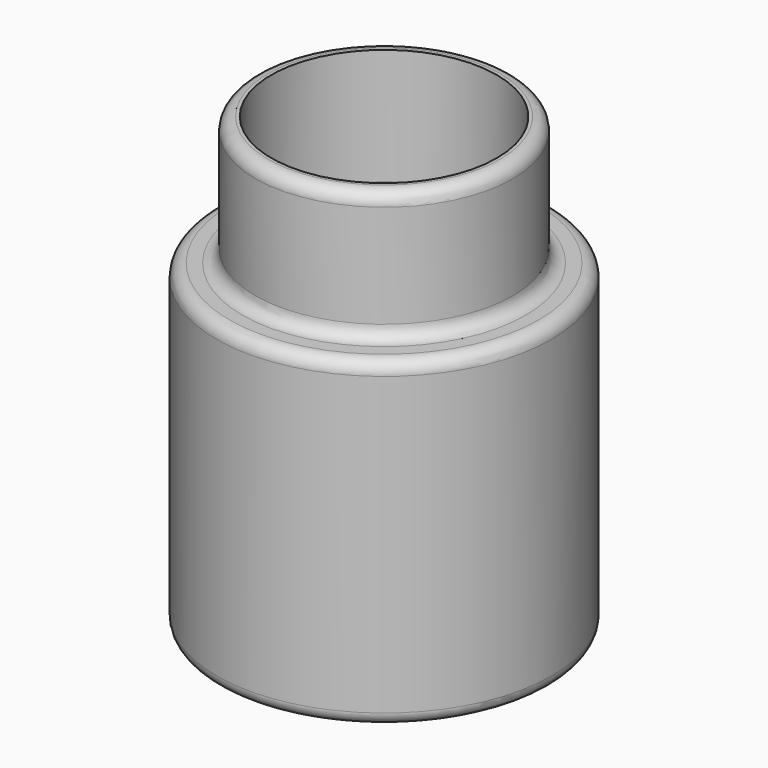
from build123d import *

# Parameters (mm, degrees)
F0_R     = 66.04
F1_DEPTH = 127
F2_R     = 5.08
F3_R     = 50.8
F3_R_2   = 44.45
F4_DEPTH = 50.8
F5_R     = 5.08
F6_T     = 2.54


# Not quite as in the source:
# - a shell that OpenCascade refuses in one call is made with other operations: the cavity is built on its own and cut out


with BuildPart() as f1:
    # F0 (on Top) → F1 (new body)
    with BuildSketch(Plane.XY):
        Circle(F0_R)
    extrude(amount=F1_DEPTH)

    # F2
    f2_edges = [f1.edges().sort_by_distance(p)[0] for p in [
        (-66.04, 0, 127),
        (-66.04, 0, 0),
    ]]
    fillet(f2_edges, radius=F2_R)

    # F3 (on face) → F4 (join)
    with BuildSketch(Plane.XY.offset(127)):
        Circle(F3_R)
        Circle(F3_R_2, mode=Mode.SUBTRACT)
    extrude(amount=F4_DEPTH)

    # F5
    f5_edges = [f1.edges().sort_by_distance(p)[0] for p in [
        (50.8, 0, 152.4),
        (-50.8, 0, 127),
        (-50.8, 0, 177.8),
        (-44.45, 0, 127),
    ]]
    fillet(f5_edges, radius=F5_R)

    # F6: shell of thickness 2.54, made by hand


with BuildPart() as f6_core1:
    # F6_t2: copy of F1
    add(f1.part)

    # the walls: a layer under each face that stays
    f6_faces = [f6_core1.faces().sort_by_distance(p)[0] for p in [
        (-40.64, -40.64, 127),
        (-52.2878975516, 0, 128.4878975516),
        (-64.5521024484, 0, 125.5121024484),
        (-50.8, 0, 152.4),
        (-66.04, 0, 63.5),
        (-49.3121024484, 0, 176.3121024484),
        (-64.5521024484, 0, 1.4878975516),
        (40.005, -22.0133333333, 177.8),
        (0, 0, 0),
        (-44.45, 0, 154.94),
        (-42.9621024484, 0, 128.4878975516),
    ]]
    thicken(f6_faces, amount=-F6_T, mode=Mode.SUBTRACT)


with BuildPart() as f1_1:
    add(f1.part)

    # what is left inside the walls is the cavity
    f6_cavity = [f6_core1.part.solids().sort_by_distance(p)[0] for p in [
        (-63.4746, 0, 82.973333),
    ]]
    add(f6_cavity, mode=Mode.SUBTRACT)


solid = f1_1.part
